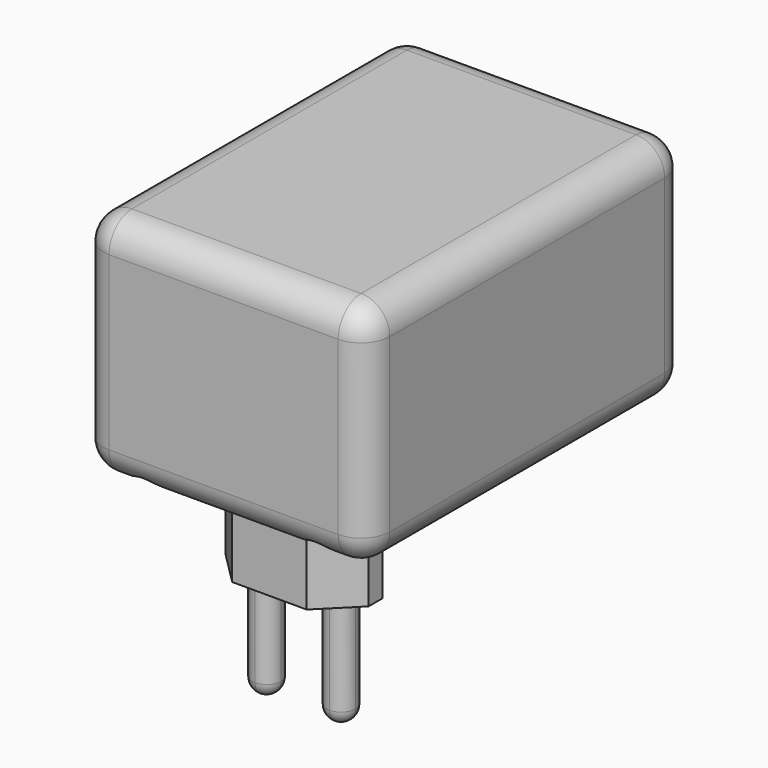
from build123d import *

# Parameters (mm, degrees)
F0_W          = 50
F0_H          = 70
F1_DEPTH      = 40
F3_DEPTH      = 15
F4_SIZE       = 6
F6_DEPTH      = 20
F7_DEPTH      = 20
F8_R          = 2.5
F10_DEPTH     = 10
F12_DEPTH     = 8
F13_T1_DEPTH  = 60
F13_T3_DEPTH  = 30
F13_T5_DEPTH  = 29.6276373277
F13_T7_DEPTH  = 29.6276373277
F13_T9_DEPTH  = 40
F13_S13_W     = 5
F13_S13_H     = 5
F13_T14_DEPTH = 5
F13_S19_W     = 5
F13_S19_H     = 5
F13_T20_DEPTH = 5
F13_S25_W     = 5
F13_S25_H     = 5
F13_T26_DEPTH = 5
F13_S31_W     = 5
F13_S31_H     = 5
F13_T32_DEPTH = 5
F13_S37_W     = 5
F13_S37_H     = 5
F13_T38_DEPTH = 5
F13_S43_W     = 5
F13_S43_H     = 5
F13_T44_DEPTH = 5
F13_S49_W     = 5
F13_S49_H     = 5
F13_T50_DEPTH = 5
F13_S55_W     = 5
F13_S55_H     = 5
F13_T56_DEPTH = 5


# Not quite as in the source:
# - a fillet or chamfer that OpenCascade refuses, or shapes differently, is made with other operations: its cross-section is extruded or revolved along the edge and cut away or added


with BuildPart() as f1:
    # F0 (on Top) → F1 (new body)
    with BuildSketch(Plane.XY):
        Rectangle(F0_W, F0_H)
    extrude(amount=F1_DEPTH)

    # F2 (on face) → F3 (join)
    with BuildSketch(Plane(origin=(0, 0, 0), x_dir=(1, 0, 0), z_dir=(0, 0, -1))):
        Polygon((-12.5, 25), (-12.5, 20), (-12.5, 10), (12.5, 10), (12.5, 17.5), (12.5, 25), align=None)
    extrude(amount=F3_DEPTH)

    # F4
    f4_edges = [f1.edges().sort_by_distance(p)[0] for p in [
        (-12.5, -25, -7.5),
        (-12.5, -10, -7.5),
        (12.5, -10, -7.5),
        (12.5, -25, -7.5),
    ]]
    chamfer(f4_edges, length=F4_SIZE)

    # F5 (on face) → F6 (join)
    with BuildSketch(Plane(origin=(0, 0, -15), x_dir=(1, 0, 0), z_dir=(0, 0, -1))):
        with BuildLine():
            ThreePointArc((-4, 17.5), (-4.732233047, 19.267766953), (-6.5, 20))
            ThreePointArc((-6.5, 20), (-8.267766953, 15.732233047), (-4, 17.5))
        make_face()
    extrude(amount=F6_DEPTH)

    # F5 (on face) → F7 (join)
    with BuildSketch(Plane(origin=(0, 0, -15), x_dir=(1, 0, 0), z_dir=(0, 0, -1))):
        with BuildLine():
            ThreePointArc((9, 17.5), (8.267766953, 19.267766953), (6.5, 20))
            ThreePointArc((6.5, 20), (4.732233047, 15.732233047), (9, 17.5))
        make_face()
    extrude(amount=F7_DEPTH)

    # F8
    f8_edges = [f1.edges().sort_by_distance(p)[0] for p in [
        (-9, -17.5, -35),
        (4, -17.5, -35),
    ]]
    fillet(f8_edges, radius=F8_R)

    # F9 (on face) → F10 (cut)
    with BuildSketch(Plane(origin=(0, 0, 0), x_dir=(1, 0, 0), z_dir=(0, 0, -1))):
        with BuildLine():
            Line((-2.8723626723, -35), (2.8723626723, -35))
            ThreePointArc((2.8723626723, -35), (0, -29.4152137969), (-2.8723626723, -35))
        make_face()
    extrude(amount=-F10_DEPTH, mode=Mode.SUBTRACT)

    # F11 (on face) → F12 (cut)
    with BuildSketch(Plane(origin=(0, 0, 0), x_dir=(1, 0, 0), z_dir=(0, 0, -1))):
        with BuildLine():
            ThreePointArc((11, 29.8445560038), (15, 25.8445560038), (19, 29.8445560038))
            Line((19, 29.8445560038), (15, 29.8445560038))
            Line((15, 29.8445560038), (11, 29.8445560038))
        make_face()
        with BuildLine():
            Line((-15, 29.8445560038), (-11, 29.8445560038))
            ThreePointArc((-11, 29.8445560038), (-15, 33.8445560038), (-19, 29.8445560038))
            Line((-19, 29.8445560038), (-15, 29.8445560038))
        make_face()
        with BuildLine():
            ThreePointArc((-19, 29.8445560038), (-15, 25.8445560038), (-11, 29.8445560038))
            Line((-11, 29.8445560038), (-15, 29.8445560038))
            Line((-15, 29.8445560038), (-19, 29.8445560038))
        make_face()
        with BuildLine():
            Line((15, 29.8445560038), (19, 29.8445560038))
            ThreePointArc((19, 29.8445560038), (15, 33.8445560038), (11, 29.8445560038))
            Line((11, 29.8445560038), (15, 29.8445560038))
        make_face()
    extrude(amount=-F12_DEPTH, mode=Mode.SUBTRACT)

    # F13: fillet of radius 5 on 13 edges, made by hand

    # F13_s2 → F13_t1 (cut)
    with BuildSketch(Plane.XZ.offset(-30)):
        with BuildLine():
            ThreePointArc((20, 0), (23.5355339059, 1.4644660941), (25, 5))
            Line((25, 5), (25, 0))
            Line((25, 0), (20, 0))
        make_face()
        with BuildLine():
            ThreePointArc((25, 35), (23.5355339059, 38.5355339059), (20, 40))
            Line((20, 40), (25, 40))
            Line((25, 40), (25, 35))
        make_face()
        with BuildLine():
            ThreePointArc((-20, 0), (-23.5355339059, 1.4644660941), (-25, 5))
            Line((-25, 5), (-25, 0))
            Line((-25, 0), (-20, 0))
        make_face()
        with BuildLine():
            ThreePointArc((-25, 35), (-23.5355339059, 38.5355339059), (-20, 40))
            Line((-20, 40), (-25, 40))
            Line((-25, 40), (-25, 35))
        make_face()
    extrude(amount=F13_T1_DEPTH, mode=Mode.SUBTRACT)

    # F13_s4 → F13_t3 (cut)
    with BuildSketch(Plane.XY.offset(5)):
        with BuildLine():
            ThreePointArc((20, -35), (23.5355339059, -33.5355339059), (25, -30))
            Line((25, -30), (25, -35))
            Line((25, -35), (20, -35))
        make_face()
        with BuildLine():
            ThreePointArc((20, 35), (23.5355339059, 33.5355339059), (25, 30))
            Line((25, 30), (25, 35))
            Line((25, 35), (20, 35))
        make_face()
        with BuildLine():
            ThreePointArc((-25, -30), (-23.5355339059, -33.5355339059), (-20, -35))
            Line((-20, -35), (-25, -35))
            Line((-25, -35), (-25, -30))
        make_face()
        with BuildLine():
            ThreePointArc((-25, 30), (-23.5355339059, 33.5355339059), (-20, 35))
            Line((-20, 35), (-25, 35))
            Line((-25, 35), (-25, 30))
        make_face()
    extrude(amount=F13_T3_DEPTH, mode=Mode.SUBTRACT)

    # F13_s6 → F13_t5 (cut)
    with BuildSketch(Plane.YZ.offset(-9.6276373277)):
        with BuildLine():
            ThreePointArc((30, 0), (33.5355339059, 1.4644660941), (35, 5))
            Line((35, 5), (35, 0))
            Line((35, 0), (30, 0))
        make_face()
    extrude(amount=F13_T5_DEPTH, mode=Mode.SUBTRACT)

    # F13_s8 → F13_t7 (cut)
    with BuildSketch(Plane.YZ.offset(-20)):
        with BuildLine():
            ThreePointArc((30, 0), (33.5355339059, 1.4644660941), (35, 5))
            Line((35, 5), (35, 0))
            Line((35, 0), (30, 0))
        make_face()
    extrude(amount=F13_T7_DEPTH, mode=Mode.SUBTRACT)

    # F13_s10 → F13_t9 (cut)
    with BuildSketch(Plane.YZ.offset(-20)):
        with BuildLine():
            ThreePointArc((-30, 0), (-33.5355339059, 1.4644660941), (-35, 5))
            Line((-35, 5), (-35, 0))
            Line((-35, 0), (-30, 0))
        make_face()
        with BuildLine():
            ThreePointArc((-35, 35), (-33.5355339059, 38.5355339059), (-30, 40))
            Line((-30, 40), (-35, 40))
            Line((-35, 40), (-35, 35))
        make_face()
        with BuildLine():
            ThreePointArc((35, 35), (33.5355339059, 38.5355339059), (30, 40))
            Line((30, 40), (35, 40))
            Line((35, 40), (35, 35))
        make_face()
    extrude(amount=F13_T9_DEPTH, mode=Mode.SUBTRACT)


with BuildPart() as f13_tool12:
    # F13_s13 → F13_t14 (new body)
    with BuildSketch(Plane.XZ.offset(30)):
        with Locations((22.5, 2.5)):
            Rectangle(F13_S13_W, F13_S13_H)
    extrude(amount=F13_T14_DEPTH)

    # F13_s15 → F13_t16 (revolve, cut)
    with BuildSketch(Plane(origin=(20, -30, 5), x_dir=(-0.7071067812, 0, 0.7071067812), z_dir=(0.7071067812, 0, 0.7071067812))):
        with BuildLine():
            ThreePointArc((0, -5), (5, 0), (0, 5))
            Line((0, 5), (0, -5))
        make_face()
    revolve(axis=Axis((20, -30, 5), (0, -1, 0)), mode=Mode.SUBTRACT)


with BuildPart() as f1_1:
    add(f1.part)

    # F13_t11: cut F13_tool12
    add(f13_tool12.part, mode=Mode.SUBTRACT)


with BuildPart() as f13_tool18:
    # F13_s19 → F13_t20 (new body)
    with BuildSketch(Plane.YZ.offset(20)):
        with Locations((32.5, 2.5)):
            Rectangle(F13_S19_W, F13_S19_H)
    extrude(amount=F13_T20_DEPTH)

    # F13_s21 → F13_t22 (revolve, cut)
    with BuildSketch(Plane(origin=(20, 30, 5), x_dir=(0, -0.7071067812, 0.7071067812), z_dir=(0, 0.7071067812, 0.7071067812))):
        with BuildLine():
            ThreePointArc((0, -5), (5, 0), (0, 5))
            Line((0, 5), (0, -5))
        make_face()
    revolve(axis=Axis((20, 30, 5), (1, 0, 0)), mode=Mode.SUBTRACT)


with BuildPart() as f1_2:
    add(f1_1.part)

    # F13_t17: cut F13_tool18
    add(f13_tool18.part, mode=Mode.SUBTRACT)


with BuildPart() as f13_tool24:
    # F13_s25 → F13_t26 (new body)
    with BuildSketch(Plane.XZ.offset(30)):
        with Locations((22.5, 37.5)):
            Rectangle(F13_S25_W, F13_S25_H)
    extrude(amount=F13_T26_DEPTH)

    # F13_s27 → F13_t28 (revolve, cut)
    with BuildSketch(Plane(origin=(20, -30, 35), x_dir=(-0.7071067812, 0, -0.7071067812), z_dir=(-0.7071067812, 0, 0.7071067812))):
        with BuildLine():
            ThreePointArc((0, -5), (5, 0), (0, 5))
            Line((0, 5), (0, -5))
        make_face()
    revolve(axis=Axis((20, -30, 35), (0, -1, 0)), mode=Mode.SUBTRACT)


with BuildPart() as f1_3:
    add(f1_2.part)

    # F13_t23: cut F13_tool24
    add(f13_tool24.part, mode=Mode.SUBTRACT)


with BuildPart() as f13_tool30:
    # F13_s31 → F13_t32 (new body)
    with BuildSketch(Plane.YZ.offset(20)):
        with Locations((32.5, 37.5)):
            Rectangle(F13_S31_W, F13_S31_H)
    extrude(amount=F13_T32_DEPTH)

    # F13_s33 → F13_t34 (revolve, cut)
    with BuildSketch(Plane(origin=(20, 30, 35), x_dir=(0, -0.7071067812, -0.7071067812), z_dir=(0, -0.7071067812, 0.7071067812))):
        with BuildLine():
            ThreePointArc((0, -5), (5, 0), (0, 5))
            Line((0, 5), (0, -5))
        make_face()
    revolve(axis=Axis((20, 30, 35), (1, 0, 0)), mode=Mode.SUBTRACT)


with BuildPart() as f1_4:
    add(f1_3.part)

    # F13_t29: cut F13_tool30
    add(f13_tool30.part, mode=Mode.SUBTRACT)


with BuildPart() as f13_tool36:
    # F13_s37 → F13_t38 (new body)
    with BuildSketch(Plane.XY.offset(5)):
        with Locations((-22.5, 32.5)):
            Rectangle(F13_S37_W, F13_S37_H)
    extrude(amount=-F13_T38_DEPTH)

    # F13_s39 → F13_t40 (revolve, cut)
    with BuildSketch(Plane(origin=(-20, 30, 5), x_dir=(0.7071067812, -0.7071067812, 0), z_dir=(0.7071067812, 0.7071067812, 0))):
        with BuildLine():
            ThreePointArc((0, -5), (5, 0), (0, 5))
            Line((0, 5), (0, -5))
        make_face()
    revolve(axis=Axis((-20, 30, 5), (0, 0, -1)), mode=Mode.SUBTRACT)


with BuildPart() as f1_5:
    add(f1_4.part)

    # F13_t35: cut F13_tool36
    add(f13_tool36.part, mode=Mode.SUBTRACT)


with BuildPart() as f13_tool42:
    # F13_s43 → F13_t44 (new body)
    with BuildSketch(Plane.XZ.offset(30)):
        with Locations((-22.5, 2.5)):
            Rectangle(F13_S43_W, F13_S43_H)
    extrude(amount=F13_T44_DEPTH)

    # F13_s45 → F13_t46 (revolve, cut)
    with BuildSketch(Plane(origin=(-20, -30, 5), x_dir=(0.7071067812, 0, 0.7071067812), z_dir=(0.7071067812, 0, -0.7071067812))):
        with BuildLine():
            ThreePointArc((0, -5), (5, 0), (0, 5))
            Line((0, 5), (0, -5))
        make_face()
    revolve(axis=Axis((-20, -30, 5), (0, -1, 0)), mode=Mode.SUBTRACT)


with BuildPart() as f1_6:
    add(f1_5.part)

    # F13_t41: cut F13_tool42
    add(f13_tool42.part, mode=Mode.SUBTRACT)


with BuildPart() as f13_tool48:
    # F13_s49 → F13_t50 (new body)
    with BuildSketch(Plane.XZ.offset(30)):
        with Locations((-22.5, 37.5)):
            Rectangle(F13_S49_W, F13_S49_H)
    extrude(amount=F13_T50_DEPTH)

    # F13_s51 → F13_t52 (revolve, cut)
    with BuildSketch(Plane(origin=(-20, -30, 35), x_dir=(0.7071067812, 0, -0.7071067812), z_dir=(-0.7071067812, 0, -0.7071067812))):
        with BuildLine():
            ThreePointArc((0, -5), (5, 0), (0, 5))
            Line((0, 5), (0, -5))
        make_face()
    revolve(axis=Axis((-20, -30, 35), (0, -1, 0)), mode=Mode.SUBTRACT)


with BuildPart() as f1_7:
    add(f1_6.part)

    # F13_t47: cut F13_tool48
    add(f13_tool48.part, mode=Mode.SUBTRACT)


with BuildPart() as f13_tool54:
    # F13_s55 → F13_t56 (new body)
    with BuildSketch(Plane.XY.offset(35)):
        with Locations((-22.5, 32.5)):
            Rectangle(F13_S55_W, F13_S55_H)
    extrude(amount=F13_T56_DEPTH)

    # F13_s57 → F13_t58 (revolve, cut)
    with BuildSketch(Plane(origin=(-20, 30, 35), x_dir=(0.7071067812, -0.7071067812, 0), z_dir=(-0.7071067812, -0.7071067812, 0))):
        with BuildLine():
            ThreePointArc((0, -5), (5, 0), (0, 5))
            Line((0, 5), (0, -5))
        make_face()
    revolve(axis=Axis((-20, 30, 35), (0, 0, 1)), mode=Mode.SUBTRACT)


with BuildPart() as f1_8:
    add(f1_7.part)

    # F13_t53: cut F13_tool54
    add(f13_tool54.part, mode=Mode.SUBTRACT)


solid = f1_8.part
